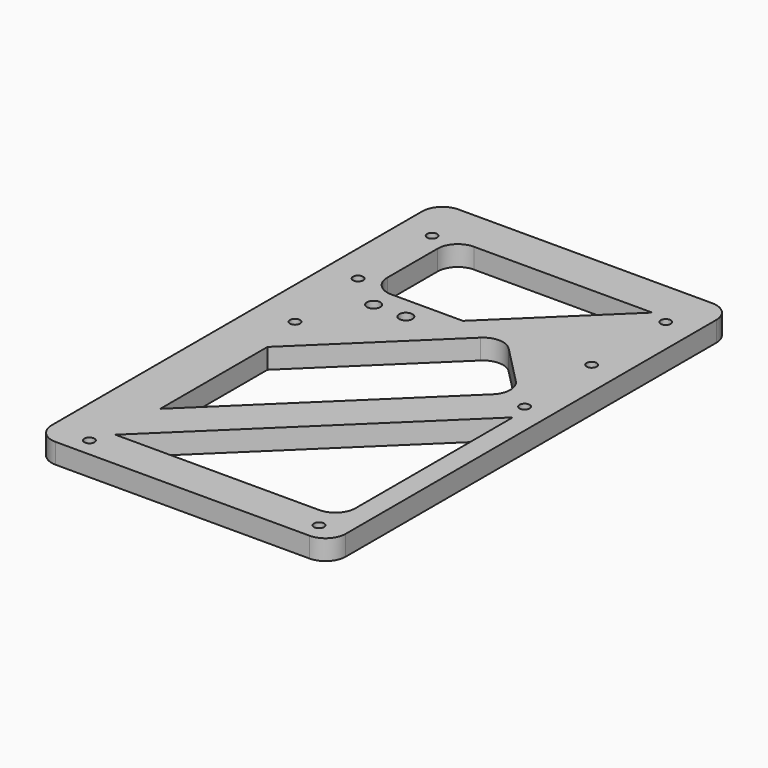
from build123d import *

# Parameters (mm, degrees)
F0_W     = 73
F0_H     = 125
F1_DEPTH = 5
F2_D     = 2.5
F3_D     = 3.3
F4_D     = 2.5
F6_DEPTH = 25
F7_R     = 5


# Not quite as in the source:
# - a feature names something its author has since deleted; it is built from what else it names


with BuildPart() as f1:
    # F0 (on Top) → F1 (new body)
    with BuildSketch(Plane.XY):
        with Locations((-1.7126457989, 26.0309018195)):
            Rectangle(F0_W, F0_H)
    extrude(amount=F1_DEPTH)

    # F2 (through all)
    with Locations(Plane(origin=(0, 0, 0), x_dir=(1, 0, 0), z_dir=(0, 0, -1))):
        with Locations((-30.3091388196, -76.7177641392), (27.6908611804, -76.7177641392), (27.6908611804, -53.7177641392), (-30.3091388196, -53.7177641392)):
            Hole(F2_D / 2)

    # F3 (through all)
    with Locations(Plane(origin=(0, 0, 0), x_dir=(1, 0, 0), z_dir=(0, 0, -1))):
        with Locations((-21.0855398327, -47.0293052495), (-13.0855398327, -47.0293052495)):
            Hole(F3_D / 2)

    # F4 (through all)
    with Locations(Plane(origin=(0, 0, 0), x_dir=(1, 0, 0), z_dir=(0, 0, -1))):
        with Locations((-28.5, -31.9), (28.5, -31.9), (28.5, 31.9), (-28.5, 31.9)):
            Hole(F4_D / 2)

    # F5 (on face) → F6 (cut)
    with BuildSketch(Plane.XY.offset(5)):
        Polygon((24.0503107939, 35.5483236554), (7.3111363315, 52.6231595762), (-26.0799791984, 20.3202102417), (-26.0799791984, -12.9482956412), align=None)
        Polygon((29.5474557331, 26.9350063375), (-26.0799791984, -26.8796142191), (29.5474557331, -26.8796142191), align=None)
        Polygon((-3.3391041424, 52.5376833975), (23.1605084746, 78.173713526), (-26.1079283048, 78.173713526), (-26.1079283048, 52.5376833975), align=None)
    extrude(amount=-F6_DEPTH, mode=Mode.SUBTRACT)

    # F7
    f7_edges = [f1.edges().sort_by_distance(p)[0] for p in [
        (-38.212646, 88.530902, 2.5),
        (34.787354, 88.530902, 2.5),
        (34.787354, -36.469098, 2.5),
        (-38.212646, -36.469098, 2.5),
        (-26.107928, 52.537683, 2.5),
        (-26.107928, 78.173714, 2.5),
        (24.050311, 35.548324, 2.5),
        (7.311136, 52.62316, 2.5),
        (29.547456, -26.879614, 2.5),
    ]]
    fillet(f7_edges, radius=F7_R)


solid = f1.part
